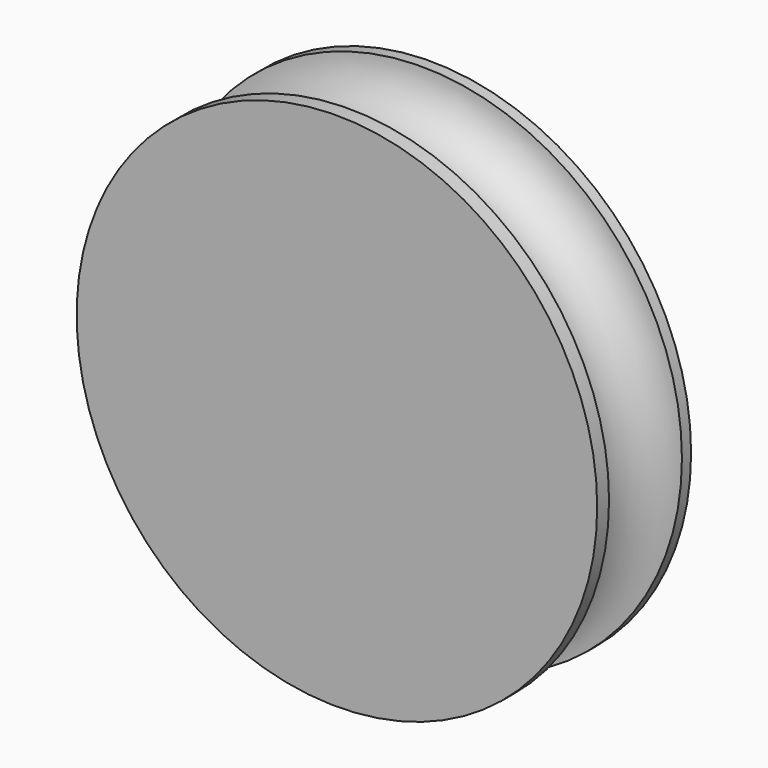
from build123d import *


# Not quite as in the source:
# - the program builds the solid bodies; features that only make, move or delete a surface that nothing else refers to are left out


with BuildPart() as f1:
    # F0 (on Top) → F1 (revolve)
    with BuildSketch(Plane.XY):
        with BuildLine():
            Line((27.0002, 5.5631161949), (1.6002, 5.5631161949))
            Line((1.6002, 5.5631161949), (1.6002, -5.8887377381))
            Line((1.6002, -5.8887377381), (27.0002, -5.8887377381))
            Line((27.0002, -5.8887377381), (27.0002, -4.445))
            ThreePointArc((27.0002, -4.445), (22.5552, 0), (27.0002, 4.445))
            Line((27.0002, 4.445), (27.0002, 5.5631161949))
        make_face()
    revolve(axis=Axis((1.6002, -0.1628107716, 0), (0, 1, 0)))


solid = f1.part
